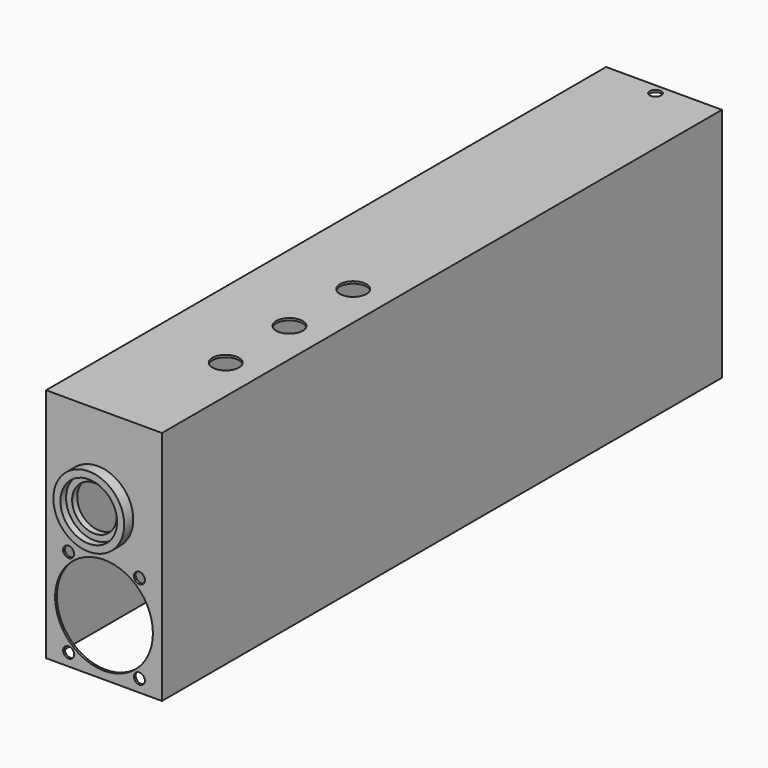
from build123d import *

# Parameters (mm, degrees)
F1_DEPTH      = 394
F2_W          = 65.42
F2_H          = 133.21
F3_DEPTH      = 1.21
F4_R          = 27.6
F5_DEPTH      = 395.211
F6_R          = 12.6
F7_DEPTH      = 395.211
F7_DEPTH_BACK = 628
F8_R          = 20
F8_R_2        = 12.6
F9_DEPTH      = 6.4
F11_R         = 7.5
F12_DEPTH     = 133.211
F13_R         = 3.25
F14_DEPTH     = 25
F10_R         = 16
F15_DEPTH     = 4
F16_R         = 3.1
F17_DEPTH     = 395.211


# Not quite as in the source:
# - an extrude ends at something that could not be found from the text; its depth is read off the source's solid


with BuildPart() as f1:
    # F0 (on Front) → F1 (new body)
    with BuildSketch(Plane.XZ):
        Polygon((-31.5, 132), (0, 132), (31.5, 132), (31.5, 0), (32.71, 0), (32.71, 133.21), (0, 133.21), (-32.71, 133.21), (-32.71, 0), (-31.5, 0), align=None)
    extrude(amount=-F1_DEPTH)

    # F2 (on face) → F3 (join)
    with BuildSketch(Plane.XZ):
        with Locations((0, 66.605)):
            Rectangle(F2_W, F2_H)
    extrude(amount=F3_DEPTH)

    # F4 (on face) → F5 (cut, through all)
    with BuildSketch(Plane.XZ.offset(1.21)):
        with Locations((0, 32)):
            Circle(F4_R)
    extrude(amount=-F5_DEPTH, mode=Mode.SUBTRACT)

    # F6 (on face) → F7 (cut, two sides)
    with BuildSketch(Plane.XZ.offset(1.21)) as f7_sk:
        with Locations((-3.5, 85)):
            Circle(F6_R)
    extrude(amount=-F7_DEPTH, mode=Mode.SUBTRACT)
    extrude(f7_sk.sketch, amount=F7_DEPTH_BACK, mode=Mode.SUBTRACT)

    # F8 (on face) → F9 (join)
    with BuildSketch(Plane.XZ.offset(1.21)):
        with Locations((-3.5, 85)):
            Circle(F8_R)
        with Locations((-3.5, 85)):
            Circle(F8_R_2, mode=Mode.SUBTRACT)
    extrude(amount=F9_DEPTH)

    # F11 (on face) → F12 (cut, through all)
    with BuildSketch(Plane.XY.offset(133.21)):
        with Locations((12.71, 68.79)):
            Circle(F11_R)
        with Locations((12.71, 113.79)):
            Circle(F11_R)
        with Locations((12.71, 158.79)):
            Circle(F11_R)
    extrude(amount=-F12_DEPTH, mode=Mode.SUBTRACT)

    # F13 (on face) → F14 (cut)
    with BuildSketch(Plane.XY.offset(133.21)):
        with Locations((0, 388)):
            Circle(F13_R)
    extrude(amount=-F14_DEPTH, mode=Mode.SUBTRACT)

    # F10 (on face) → F15 (cut)
    with BuildSketch(Plane.XZ.offset(7.61)):
        with Locations((-3.5, 85)):
            Circle(F10_R)
    extrude(amount=-F15_DEPTH, mode=Mode.SUBTRACT)

    # F16 (on face) → F17 (cut, through all)
    with BuildSketch(Plane.XZ.offset(1.21)):
        with Locations((20, 57)):
            Circle(F16_R)
        with Locations((-20, 57)):
            Circle(F16_R)
        with Locations((-20, 7)):
            Circle(F16_R)
        with Locations((20, 7)):
            Circle(F16_R)
    extrude(amount=-F17_DEPTH, mode=Mode.SUBTRACT)


solid = f1.part
